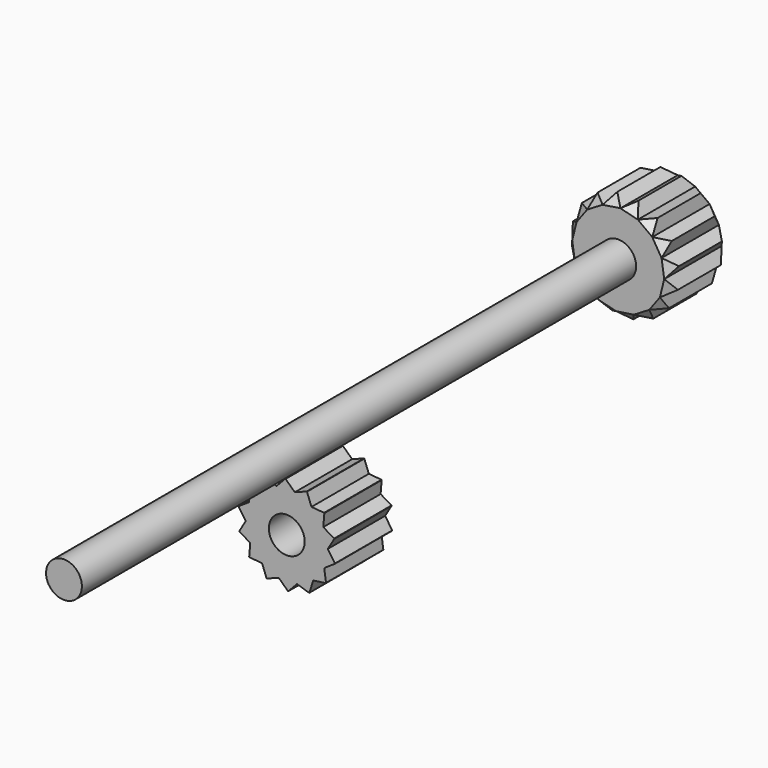
from build123d import *

# Parameters (mm, degrees)
F1_DEPTH      = 9.525
F2_DEPTH      = 1.1938
F3_DEPTH      = 1.1938
F4_DEPTH      = 1.1938
F5_DEPTH      = 1.1938
F6_DEPTH      = 1.1938
F7_DEPTH      = 1.1938
F8_DEPTH      = 1.1938
F9_DEPTH      = 1.1938
F10_DEPTH     = 1.1938
F11_DEPTH     = 1.1938
F12_DEPTH     = 1.1938
F13_DEPTH     = 1.1938
F14_DEPTH     = 1.1938
F15_DEPTH     = 1.1938
F16_SIZE      = 1.1937
F17_D         = 4.7625
F18_R         = 2.38125
F19_DEPTH     = 9.525
F20_DEPTH     = 1.1938
F21_DEPTH     = 1.1938
F22_DEPTH     = 1.1938
F23_DEPTH     = 1.1938
F24_DEPTH     = 1.1938
F25_DEPTH     = 1.1938
F26_DEPTH     = 1.1938
F27_DEPTH     = 1.1938
F28_SIZE      = 1.19379
F29_DEPTH     = 1.1938
F30_DEPTH     = 1.1938
F31_DEPTH     = 1.1938
F32_DEPTH     = 1.1938
F33_DEPTH     = 1.1938
F34_DEPTH     = 1.1938
F35_DEPTH     = 1.1938
F36_DEPTH     = 1.1938
F37_T1_DEPTH  = 8.5277503021
F37_T3_DEPTH  = 8.5277503021
F37_T5_DEPTH  = 8.5277503021
F37_T7_DEPTH  = 8.5277503021
F37_T9_DEPTH  = 8.5277503021
F37_T11_DEPTH = 8.5277503021
F37_T13_DEPTH = 8.5277503021
F37_T15_DEPTH = 8.5277503021
F37_T20_DEPTH = 15.6651503021
F37_T25_DEPTH = 15.6651503021
F37_T30_DEPTH = 15.6651503021
F37_T35_DEPTH = 15.6651503021
F37_T40_DEPTH = 15.6651503021
F37_T45_DEPTH = 15.6651503021
F37_T50_DEPTH = 15.6651503021
F37_T55_DEPTH = 15.6651503021
F37_T60_DEPTH = 15.6651503021
F37_T65_DEPTH = 15.6651503021
F37_T70_DEPTH = 15.6651503021
F37_T75_DEPTH = 15.6651503021
F37_T80_DEPTH = 15.6651503021
F37_T85_DEPTH = 15.6651503021
F37_T90_DEPTH = 15.6651503021
F37_T95_DEPTH = 15.6651503021
F38_DEPTH     = 101.6


# Not quite as in the source:
# - a fillet or chamfer that OpenCascade refuses, or shapes differently, is made with other operations: its cross-section is extruded or revolved along the edge and cut away or added
# - a fillet or chamfer is up to 0.001 mm smaller than in the source, because OpenCascade refuses the exact size


with BuildPart() as f1:
    # F0 (on Front) → F1 (new body)
    with BuildSketch(Plane.XZ):
        Polygon((3.5186572194, -4.1725797324), (4.9806151076, -2.2326762867), (5.4561010905, 0.1494360796), (4.8509393377, 2.5019507976), (3.2849895562, 4.3589234757), (1.0684073054, 5.3525579008), (-1.3597861155, 5.2860525888), (-3.5186572194, 4.1725797324), (-4.9806151076, 2.2326762867), (-5.4561010905, -0.1494360796), (-4.8509393377, -2.5019507976), (-3.2849895562, -4.3589234757), (-1.0684073054, -5.3525579008), (1.3597861155, -5.2860525888), align=None)
    extrude(amount=F1_DEPTH)

    # F2 (add): a face of the model
    f2_faces = [f1.faces().sort_by_distance(p)[0] for p in [
        (5.1535202141, -4.7625, 1.3256934386),
    ]]
    extrude(f2_faces, amount=F2_DEPTH)

    # F3 (add): a face of the model
    f3_faces = [f1.faces().sort_by_distance(p)[0] for p in [
        (5.218358099, -4.7625, -1.0416201036),
    ]]
    extrude(f3_faces, amount=F3_DEPTH)

    # F4 (add): a face of the model
    f4_faces = [f1.faces().sort_by_distance(p)[0] for p in [
        (4.2496361635, -4.7625, -3.2026280096),
    ]]
    extrude(f4_faces, amount=F4_DEPTH)

    # F5 (add): a face of the model
    f5_faces = [f1.faces().sort_by_distance(p)[0] for p in [
        (4.0679644469, -4.7625, 3.4304371366),
    ]]
    extrude(f5_faces, amount=F5_DEPTH)

    # F6 (add): a face of the model
    f6_faces = [f1.faces().sort_by_distance(p)[0] for p in [
        (2.1766984308, -4.7625, 4.8557406882),
    ]]
    extrude(f6_faces, amount=F6_DEPTH)

    # F7 (add): a face of the model
    f7_faces = [f1.faces().sort_by_distance(p)[0] for p in [
        (-0.1456894051, -4.7625, 5.3193052448),
    ]]
    extrude(f7_faces, amount=F7_DEPTH)

    # F8 (add): a face of the model
    f8_faces = [f1.faces().sort_by_distance(p)[0] for p in [
        (-2.4392216675, -4.7625, 4.7293161606),
    ]]
    extrude(f8_faces, amount=F8_DEPTH)

    # F9 (add): a face of the model
    f9_faces = [f1.faces().sort_by_distance(p)[0] for p in [
        (-4.2496361635, -4.7625, 3.2026280096),
    ]]
    extrude(f9_faces, amount=F9_DEPTH)

    # F10 (add): a face of the model
    f10_faces = [f1.faces().sort_by_distance(p)[0] for p in [
        (-5.218358099, -4.7625, 1.0416201036),
    ]]
    extrude(f10_faces, amount=F10_DEPTH)

    # F11 (add): a face of the model
    f11_faces = [f1.faces().sort_by_distance(p)[0] for p in [
        (-5.1535202141, -4.7625, -1.3256934386),
    ]]
    extrude(f11_faces, amount=F11_DEPTH)

    # F12 (add): a face of the model
    f12_faces = [f1.faces().sort_by_distance(p)[0] for p in [
        (-4.0679644469, -4.7625, -3.4304371366),
    ]]
    extrude(f12_faces, amount=F12_DEPTH)

    # F13 (add): a face of the model
    f13_faces = [f1.faces().sort_by_distance(p)[0] for p in [
        (-2.1766984308, -4.7625, -4.8557406882),
    ]]
    extrude(f13_faces, amount=F13_DEPTH)

    # F14 (add): a face of the model
    f14_faces = [f1.faces().sort_by_distance(p)[0] for p in [
        (0.1456894051, -4.7625, -5.3193052448),
    ]]
    extrude(f14_faces, amount=F14_DEPTH)

    # F15 (add): a face of the model
    f15_faces = [f1.faces().sort_by_distance(p)[0] for p in [
        (2.4392216675, -4.7625, -4.7293161606),
    ]]
    extrude(f15_faces, amount=F15_DEPTH)

    # F16 (size 1.1938 in the source; OpenCascade refuses exactly that, so slightly less here)
    f16_edges = [f1.edges().sort_by_distance(p)[0] for p in [
        (4.472036, -4.7625, -4.891069),
        (4.065881, -4.7625, -5.233572),
        (1.90701, -4.7625, -6.347045),
        (5.933994, -4.7625, -2.951166),
        (6.151321, -4.7625, -2.466357),
        (6.626807, -4.7625, -0.084245),
        (6.612261, -4.7625, 0.446847),
        (5.763561, -4.7625, 3.271548),
        (6.007099, -4.7625, 2.799362),
        (4.197612, -4.7625, 5.12852),
        (3.773318, -4.7625, 5.448278),
        (1.556736, -4.7625, 6.441913),
        (1.035723, -4.7625, 6.54591),
        (-1.90701, -4.7625, 6.347045),
        (-1.392471, -4.7625, 6.479405),
        (-4.065881, -4.7625, 5.233572),
        (-4.472036, -4.7625, 4.891069),
        (-6.151321, -4.7625, 2.466357),
        (-5.933994, -4.7625, 2.951166),
        (-6.626807, -4.7625, 0.084245),
        (-6.612261, -4.7625, -0.446847),
        (-6.007099, -4.7625, -2.799362),
        (-5.763561, -4.7625, -3.271548),
        (-3.773318, -4.7625, -5.448278),
        (-4.197612, -4.7625, -5.12852),
        (-1.556736, -4.7625, -6.441913),
        (-1.035723, -4.7625, -6.54591),
        (1.392471, -4.7625, -6.479405),
    ]]
    chamfer(f16_edges, length=F16_SIZE)

    # F17 (through all)
    with Locations(Plane(origin=(0, 0, 0), x_dir=(1, 0, 0), z_dir=(0, 1, 0))):
        with Locations((0, 0)):
            Hole(F17_D / 2)


with BuildPart() as f19:
    # F18 (on Front) → F19 (new body)
    with BuildSketch(Plane.XZ):
        Polygon((49.5876813653, 43.9301886246), (50.1632868744, 46.2473662306), (49.8083315434, 48.6084338859), (48.5768541037, 50.6539404431), (46.6563358322, 52.0724760714), (44.3391582262, 52.6480815805), (41.9780905708, 52.2931262495), (39.9325840136, 51.0616488098), (38.5140483853, 49.1411305383), (37.9384428762, 46.8239529323), (38.2933982073, 44.4628852769), (39.5248756469, 42.4173787197), (41.4453939184, 40.9988430914), (43.7625715245, 40.4232375823), (46.1236391798, 40.7781929134), (48.169145737, 42.009670353), align=None)
        with Locations((44.0508648753, 46.5356595814)):
            Circle(F18_R, mode=Mode.SUBTRACT)
    extrude(amount=F19_DEPTH)

    # F20 (add): a face of the model
    f20_faces = [f19.faces().sort_by_distance(p)[0] for p in [
        (47.1463924584, -4.7625, 41.3939316332),
    ]]
    extrude(f20_faces, amount=F20_DEPTH)

    # F21 (add): a face of the model
    f21_faces = [f19.faces().sort_by_distance(p)[0] for p in [
        (42.6039827215, -4.7625, 40.7110403369),
    ]]
    extrude(f21_faces, amount=F21_DEPTH)

    # F22 (add): a face of the model
    f22_faces = [f19.faces().sort_by_distance(p)[0] for p in [
        (38.9091369271, -4.7625, 43.4401319983),
    ]]
    extrude(f22_faces, amount=F22_DEPTH)

    # F23 (add): a face of the model
    f23_faces = [f19.faces().sort_by_distance(p)[0] for p in [
        (38.2262456308, -4.7625, 47.9825417353),
    ]]
    extrude(f23_faces, amount=F23_DEPTH)

    # F24 (add): a face of the model
    f24_faces = [f19.faces().sort_by_distance(p)[0] for p in [
        (40.9553372922, -4.7625, 51.6773875296),
    ]]
    extrude(f24_faces, amount=F24_DEPTH)

    # F25 (add): a face of the model
    f25_faces = [f19.faces().sort_by_distance(p)[0] for p in [
        (45.4977470292, -4.7625, 52.360278826),
    ]]
    extrude(f25_faces, amount=F25_DEPTH)

    # F26 (add): a face of the model
    f26_faces = [f19.faces().sort_by_distance(p)[0] for p in [
        (49.1925928235, -4.7625, 49.6311871645),
    ]]
    extrude(f26_faces, amount=F26_DEPTH)

    # F27 (add): a face of the model
    f27_faces = [f19.faces().sort_by_distance(p)[0] for p in [
        (49.8754841199, -4.7625, 45.0887774276),
    ]]
    extrude(f27_faces, amount=F27_DEPTH)

    # F28 (size 1.1938 in the source; OpenCascade refuses exactly that, so slightly less here)
    f28_edges = [f19.edges().sort_by_distance(p)[0] for p in [
        (50.831085, -4.7625, 49.224173),
        (49.599607, -4.7625, 51.269679),
        (50.215346, 0, 50.246926),
        (50.215346, -9.525, 50.246926),
        (46.944139, -4.7625, 53.231065),
        (44.626961, -4.7625, 53.80667),
        (45.78555, 0, 53.518868),
        (45.78555, -9.525, 53.518868),
        (50.74627, -4.7625, 43.642386),
        (51.321876, -4.7625, 45.959563),
        (51.034073, 0, 44.800975),
        (51.034073, -9.525, 44.800975),
        (46.739378, -4.7625, 39.75544),
        (48.784884, -4.7625, 40.986917),
        (47.762131, 0, 40.371178),
        (47.762131, -9.525, 40.371178),
        (41.157591, -4.7625, 39.840254),
        (43.474769, -4.7625, 39.264649),
        (42.31618, 0, 39.552452),
        (42.31618, -9.525, 39.552452),
        (37.270645, -4.7625, 43.847147),
        (38.502122, -4.7625, 41.80164),
        (37.886384, 0, 42.824393),
        (37.886384, -9.525, 42.824393),
        (37.35546, -4.7625, 49.428933),
        (36.779854, -4.7625, 47.111756),
        (37.067657, 0, 48.270344),
        (37.067657, -9.525, 48.270344),
        (41.362352, -4.7625, 53.31588),
        (39.316845, -4.7625, 52.084402),
        (40.339599, 0, 52.700141),
        (40.339599, -9.525, 52.700141),
    ]]
    chamfer(f28_edges, length=F28_SIZE)

    # F29 (add): a face of the model
    f29_faces = [f19.faces().sort_by_distance(p)[0] for p in [
        (39.2233161995, -4.7625, 50.101389674),
    ]]
    extrude(f29_faces, amount=F29_DEPTH)

    # F30 (add): a face of the model
    f30_faces = [f19.faces().sort_by_distance(p)[0] for p in [
        (43.1586243985, -4.7625, 52.470603915),
    ]]
    extrude(f30_faces, amount=F30_DEPTH)

    # F31 (add): a face of the model
    f31_faces = [f19.faces().sort_by_distance(p)[0] for p in [
        (47.6165949679, -4.7625, 51.3632082573),
    ]]
    extrude(f31_faces, amount=F31_DEPTH)

    # F32 (add): a face of the model
    f32_faces = [f19.faces().sort_by_distance(p)[0] for p in [
        (49.9858092089, -4.7625, 47.4279000582),
    ]]
    extrude(f32_faces, amount=F32_DEPTH)

    # F33 (add): a face of the model
    f33_faces = [f19.faces().sort_by_distance(p)[0] for p in [
        (48.8784135512, -4.7625, 42.9699294888),
    ]]
    extrude(f33_faces, amount=F33_DEPTH)

    # F34 (add): a face of the model
    f34_faces = [f19.faces().sort_by_distance(p)[0] for p in [
        (44.9431053521, -4.7625, 40.6007152479),
    ]]
    extrude(f34_faces, amount=F34_DEPTH)

    # F35 (add): a face of the model
    f35_faces = [f19.faces().sort_by_distance(p)[0] for p in [
        (40.4851347827, -4.7625, 41.7081109056),
    ]]
    extrude(f35_faces, amount=F35_DEPTH)

    # F36 (add): a face of the model
    f36_faces = [f19.faces().sort_by_distance(p)[0] for p in [
        (38.1159205417, -4.7625, 45.6434191046),
    ]]
    extrude(f36_faces, amount=F36_DEPTH)

    # F37: chamfer of 1.1938 on 32 edges, made by hand

    # F37_s2 → F37_t1 (cut)
    with BuildSketch(Plane(origin=(-6.5016963168, 0, 43.2475400037), x_dir=(0, 1, 0), z_dir=(0.1486661631, 0, -0.9888874415))):
        Polygon((0, 44.4779871341), (-1.1938, 43.2841871341), (0, 43.2841871341), align=None)
        Polygon((-9.525, 44.4779871341), (-8.3312, 43.2841871341), (-9.525, 43.2841871341), align=None)
    extrude(amount=F37_T1_DEPTH, mode=Mode.SUBTRACT)

    # F37_s4 → F37_t3 (cut)
    with BuildSketch(Plane(origin=(40.3219298474, 0, 54.5908058057), x_dir=(0, 1, 0), z_dir=(-0.5941261636, 0, -0.8043718678))):
        Polygon((0, 1.7835856714), (-1.1938, 0.5897856714), (0, 0.5897856714), align=None)
        Polygon((-8.3312, 0.5897856714), (-9.525, 1.7835856714), (-9.525, 0.5897856714), align=None)
    extrude(amount=F37_T3_DEPTH, mode=Mode.SUBTRACT)

    # F37_s6 → F37_t5 (cut)
    with BuildSketch(Plane(origin=(2.8324735945, 0, -2.0921252194), x_dir=(0, 1, 0), z_dir=(0.8043718678, 0, -0.5941261636))):
        Polygon((0, 57.6021088837), (-1.1938, 56.4083088837), (0, 56.4083088837), align=None)
        Polygon((-8.3312, 56.4083088837), (-9.525, 57.6021088837), (-9.525, 56.4083088837), align=None)
    extrude(amount=F37_T5_DEPTH, mode=Mode.SUBTRACT)

    # F37_s8 → F37_t7 (cut)
    with BuildSketch(Plane(origin=(45.7021746445, 0, 6.8707182081), x_dir=(0, 1, 0), z_dir=(0.9888874415, 0, 0.1486661631))):
        Polygon((0, 33.4680183936), (-1.1938, 32.2742183936), (0, 32.2742183936), align=None)
        Polygon((-8.3312, 32.2742183936), (-9.525, 33.4680183936), (-9.525, 32.2742183936), align=None)
    extrude(amount=F37_T7_DEPTH, mode=Mode.SUBTRACT)

    # F37_s10 → F37_t9 (cut)
    with BuildSketch(Plane(origin=(54.1351598224, 0, 8.1385061254), x_dir=(0, 1, 0), z_dir=(-0.9888874415, 0, -0.1486661631))):
        Polygon((0, -45.471294165), (-1.1938, -46.665094165), (0, -46.665094165), align=None)
        Polygon((-8.3312, -46.665094165), (-9.525, -45.471294165), (-9.525, -46.665094165), align=None)
    extrude(amount=F37_T9_DEPTH, mode=Mode.SUBTRACT)

    # F37_s12 → F37_t11 (cut)
    with BuildSketch(Plane(origin=(9.6919560329, 0, -7.1586847909), x_dir=(0, 1, 0), z_dir=(-0.8043718678, 0, 0.5941261636))):
        Polygon((0, -69.6053846551), (-1.1938, -70.7991846551), (0, -70.7991846551), align=None)
        Polygon((-8.3312, -70.7991846551), (-9.525, -69.6053846551), (-9.525, -70.7991846551), align=None)
    extrude(amount=F37_T11_DEPTH, mode=Mode.SUBTRACT)

    # F37_s14 → F37_t13 (cut)
    with BuildSketch(Plane(origin=(-5.2339083995, 0, 34.8145548257), x_dir=(0, 1, 0), z_dir=(-0.1486661631, 0, 0.9888874415))):
        Polygon((0, -56.4812629055), (-1.1938, -57.6750629055), (0, -57.6750629055), align=None)
        Polygon((-8.3312, -57.6750629055), (-9.525, -56.4812629055), (-9.525, -57.6750629055), align=None)
    extrude(amount=F37_T13_DEPTH, mode=Mode.SUBTRACT)

    # F37_s16 → F37_t15 (cut)
    with BuildSketch(Plane(origin=(35.2553702759, 0, 47.7313233673), x_dir=(0, 1, 0), z_dir=(0.5941261636, 0, 0.8043718678))):
        Polygon((0, -13.7868614428), (-1.1938, -14.9806614428), (0, -14.9806614428), align=None)
        Polygon((-8.3312, -14.9806614428), (-9.525, -13.7868614428), (-9.525, -14.9806614428), align=None)
    extrude(amount=F37_T15_DEPTH, mode=Mode.SUBTRACT)


with BuildPart() as f37_tool18:
    # F37_s19 → F37_t20 (new body)
    with BuildSketch(Plane.XZ.offset(-3.070075151)):
        Polygon((37.9384428762, 46.8239529323), (36.9353867141, 45.4659414391), (36.7579090486, 46.6464752667), align=None)
    extrude(amount=F37_T20_DEPTH)

    split(bisect_by=Plane(origin=(48.5362534503, 0, 29.2207819721), x_dir=(0, 1, 0), z_dir=(-0.8567207896, 0, -0.5157804656)), keep=Keep.TOP)


with BuildPart() as f19_1:
    add(f19.part)

    # F37_t17: cut F37_tool18
    add(f37_tool18.part, mode=Mode.SUBTRACT)


with BuildPart() as f37_tool23:
    # F37_s24 → F37_t25 (new body)
    with BuildSketch(Plane.XZ.offset(-3.070075151)):
        Polygon((38.2933982073, 44.4628852769), (36.9353867141, 45.4659414391), (37.1128643796, 44.2854076114), align=None)
    extrude(amount=F37_T25_DEPTH)

    split(bisect_by=Plane(origin=(25.6647692084, 0, -6.3753345912), x_dir=(0, 1, 0), z_dir=(-0.9705049447, 0, 0.2410812151)), keep=Keep.TOP)


with BuildPart() as f19_2:
    add(f19_1.part)

    # F37_t22: cut F37_tool23
    add(f37_tool23.part, mode=Mode.SUBTRACT)


with BuildPart() as f37_tool28:
    # F37_s29 → F37_t30 (new body)
    with BuildSketch(Plane.XZ.offset(-3.070075151)):
        Polygon((39.9325840136, 51.0616488098), (38.2630570637, 50.8106574882), (38.9723248779, 51.770916624), align=None)
    extrude(amount=F37_T30_DEPTH)

    split(bisect_by=Plane(origin=(25.6647692084, 0, -6.3753345912), x_dir=(0, 1, 0), z_dir=(-0.9705049447, 0, 0.2410812151)), keep=Keep.TOP)


with BuildPart() as f19_3:
    add(f19_2.part)

    # F37_t27: cut F37_tool28
    add(f37_tool28.part, mode=Mode.SUBTRACT)


with BuildPart() as f37_tool33:
    # F37_s34 → F37_t35 (new body)
    with BuildSketch(Plane.XZ.offset(-3.070075151)):
        Polygon((38.2630570637, 50.8106574882), (38.5140483853, 49.1411305383), (37.5537892496, 49.8503983525), align=None)
    extrude(amount=F37_T35_DEPTH)

    split(bisect_by=Plane(origin=(-11.4686063276, 0, 19.0495649285), x_dir=(0, 1, 0), z_dir=(-0.5157804656, 0, 0.8567207896)), keep=Keep.TOP)


with BuildPart() as f19_4:
    add(f19_3.part)

    # F37_t32: cut F37_tool33
    add(f37_tool33.part, mode=Mode.SUBTRACT)


with BuildPart() as f37_tool38:
    # F37_s39 → F37_t40 (new body)
    with BuildSketch(Plane.XZ.offset(-3.070075151)):
        Polygon((39.5248756469, 42.4173787197), (39.7758669685, 40.7478517698), (38.8156078328, 41.457119584), align=None)
    extrude(amount=F37_T40_DEPTH)

    split(bisect_by=Plane(origin=(12.2216058729, 0, 49.1997227119), x_dir=(0, 1, 0), z_dir=(-0.2410812151, 0, -0.9705049447)), keep=Keep.TOP)


with BuildPart() as f19_5:
    add(f19_4.part)

    # F37_t37: cut F37_tool38
    add(f37_tool38.part, mode=Mode.SUBTRACT)


with BuildPart() as f37_tool43:
    # F37_s44 → F37_t45 (new body)
    with BuildSketch(Plane.XZ.offset(-3.070075151)):
        Polygon((39.7758669685, 40.7478517698), (41.4453939184, 40.9988430914), (40.7361261043, 40.0385839557), align=None)
    extrude(amount=F37_T45_DEPTH)

    split(bisect_by=Plane(origin=(48.5362534503, 0, 29.2207819721), x_dir=(0, 1, 0), z_dir=(-0.8567207896, 0, -0.5157804656)), keep=Keep.TOP)


with BuildPart() as f19_6:
    add(f19_5.part)

    # F37_t42: cut F37_tool43
    add(f37_tool43.part, mode=Mode.SUBTRACT)


with BuildPart() as f37_tool48:
    # F37_s49 → F37_t50 (new body)
    with BuildSketch(Plane.XZ.offset(-3.070075151)):
        Polygon((43.7625715245, 40.4232375823), (45.1205830177, 39.4201814202), (43.94004919, 39.2427037547), align=None)
    extrude(amount=F37_T50_DEPTH)

    split(bisect_by=Plane(origin=(-6.2200758942, 0, 10.3316598567), x_dir=(0, 1, 0), z_dir=(0.5157804656, 0, -0.8567207896)), keep=Keep.TOP)


with BuildPart() as f19_7:
    add(f19_6.part)

    # F37_t47: cut F37_tool48
    add(f37_tool48.part, mode=Mode.SUBTRACT)


with BuildPart() as f37_tool53:
    # F37_s54 → F37_t55 (new body)
    with BuildSketch(Plane.XZ.offset(-3.070075151)):
        Polygon((45.1205830177, 39.4201814202), (46.1236391798, 40.7781929134), (46.3011168453, 39.5976590857), align=None)
    extrude(amount=F37_T55_DEPTH)

    split(bisect_by=Plane(origin=(12.2216058729, 0, 49.1997227119), x_dir=(0, 1, 0), z_dir=(-0.2410812151, 0, -0.9705049447)), keep=Keep.TOP)


with BuildPart() as f19_8:
    add(f19_7.part)

    # F37_t52: cut F37_tool53
    add(f37_tool53.part, mode=Mode.SUBTRACT)


with BuildPart() as f37_tool58:
    # F37_s59 → F37_t60 (new body)
    with BuildSketch(Plane.XZ.offset(-3.070075151)):
        Polygon((44.3391582262, 52.6480815805), (42.981146733, 53.6511377427), (44.1616805606, 53.8286154082), align=None)
    extrude(amount=F37_T60_DEPTH)

    split(bisect_by=Plane(origin=(-11.4686063276, 0, 19.0495649285), x_dir=(0, 1, 0), z_dir=(-0.5157804656, 0, 0.8567207896)), keep=Keep.TOP)


with BuildPart() as f19_9:
    add(f19_8.part)

    # F37_t57: cut F37_tool58
    add(f37_tool58.part, mode=Mode.SUBTRACT)


with BuildPart() as f37_tool63:
    # F37_s64 → F37_t65 (new body)
    with BuildSketch(Plane.XZ.offset(-3.070075151)):
        Polygon((42.981146733, 53.6511377427), (41.9780905708, 52.2931262495), (41.8006129053, 53.4736600771), align=None)
    extrude(amount=F37_T65_DEPTH)

    split(bisect_by=Plane(origin=(14.6748242062, 0, 59.0754839667), x_dir=(0, 1, 0), z_dir=(0.2410812151, 0, 0.9705049447)), keep=Keep.TOP)


with BuildPart() as f19_10:
    add(f19_9.part)

    # F37_t62: cut F37_tool63
    add(f37_tool63.part, mode=Mode.SUBTRACT)


with BuildPart() as f37_tool68:
    # F37_s69 → F37_t70 (new body)
    with BuildSketch(Plane.XZ.offset(-3.070075151)):
        Polygon((48.5768541037, 50.6539404431), (48.3258627821, 52.323467393), (49.2861219179, 51.6141995789), align=None)
    extrude(amount=F37_T70_DEPTH)

    split(bisect_by=Plane(origin=(14.6748242062, 0, 59.0754839667), x_dir=(0, 1, 0), z_dir=(0.2410812151, 0, 0.9705049447)), keep=Keep.TOP)


with BuildPart() as f19_11:
    add(f19_10.part)

    # F37_t67: cut F37_tool68
    add(f37_tool68.part, mode=Mode.SUBTRACT)


with BuildPart() as f37_tool73:
    # F37_s74 → F37_t75 (new body)
    with BuildSketch(Plane.XZ.offset(-3.070075151)):
        Polygon((48.3258627821, 52.323467393), (46.6563358322, 52.0724760714), (47.3656036464, 53.0327352072), align=None)
    extrude(amount=F37_T75_DEPTH)

    split(bisect_by=Plane(origin=(57.2541585222, 0, 34.4693124055), x_dir=(0, 1, 0), z_dir=(0.8567207896, 0, 0.5157804656)), keep=Keep.TOP)


with BuildPart() as f19_12:
    add(f19_11.part)

    # F37_t72: cut F37_tool73
    add(f37_tool73.part, mode=Mode.SUBTRACT)


with BuildPart() as f37_tool78:
    # F37_s79 → F37_t80 (new body)
    with BuildSketch(Plane.XZ.offset(-3.070075151)):
        Polygon((50.1632868744, 46.2473662306), (51.1663430365, 47.6053777238), (51.3438207021, 46.4248438961), align=None)
    extrude(amount=F37_T80_DEPTH)

    split(bisect_by=Plane(origin=(57.2541585222, 0, 34.4693124055), x_dir=(0, 1, 0), z_dir=(0.8567207896, 0, 0.5157804656)), keep=Keep.TOP)


with BuildPart() as f19_13:
    add(f19_12.part)

    # F37_t77: cut F37_tool78
    add(f37_tool78.part, mode=Mode.SUBTRACT)


with BuildPart() as f37_tool83:
    # F37_s84 → F37_t85 (new body)
    with BuildSketch(Plane.XZ.offset(-3.070075151)):
        Polygon((51.1663430365, 47.6053777238), (49.8083315434, 48.6084338859), (50.988865371, 48.7859115514), align=None)
    extrude(amount=F37_T85_DEPTH)

    split(bisect_by=Plane(origin=(35.5405304631, 0, -8.8285529245), x_dir=(0, 1, 0), z_dir=(0.9705049447, 0, -0.2410812151)), keep=Keep.TOP)


with BuildPart() as f19_14:
    add(f19_13.part)

    # F37_t82: cut F37_tool83
    add(f37_tool83.part, mode=Mode.SUBTRACT)


with BuildPart() as f37_tool88:
    # F37_s89 → F37_t90 (new body)
    with BuildSketch(Plane.XZ.offset(-3.070075151)):
        Polygon((48.169145737, 42.009670353), (49.8386726869, 42.2606616746), (49.1294048727, 41.3004025389), align=None)
    extrude(amount=F37_T90_DEPTH)

    split(bisect_by=Plane(origin=(35.5405304631, 0, -8.8285529245), x_dir=(0, 1, 0), z_dir=(0.9705049447, 0, -0.2410812151)), keep=Keep.TOP)


with BuildPart() as f19_15:
    add(f19_14.part)

    # F37_t87: cut F37_tool88
    add(f37_tool88.part, mode=Mode.SUBTRACT)


with BuildPart() as f37_tool93:
    # F37_s94 → F37_t95 (new body)
    with BuildSketch(Plane.XZ.offset(-3.070075151)):
        Polygon((49.8386726869, 42.2606616746), (49.5876813653, 43.9301886246), (50.5479405011, 43.2209208104), align=None)
    extrude(amount=F37_T95_DEPTH)

    split(bisect_by=Plane(origin=(-6.2200758942, 0, 10.3316598567), x_dir=(0, 1, 0), z_dir=(0.5157804656, 0, -0.8567207896)), keep=Keep.TOP)


with BuildPart() as f19_16:
    add(f19_15.part)

    # F37_t92: cut F37_tool93
    add(f37_tool93.part, mode=Mode.SUBTRACT)

    # F18 (on Front) → F38 (join)
    with BuildSketch(Plane.XZ):
        with Locations((44.0508648753, 46.5356595814)):
            Circle(F18_R)
    extrude(amount=F38_DEPTH)


solid = Compound([f1.part, f19_16.part])
